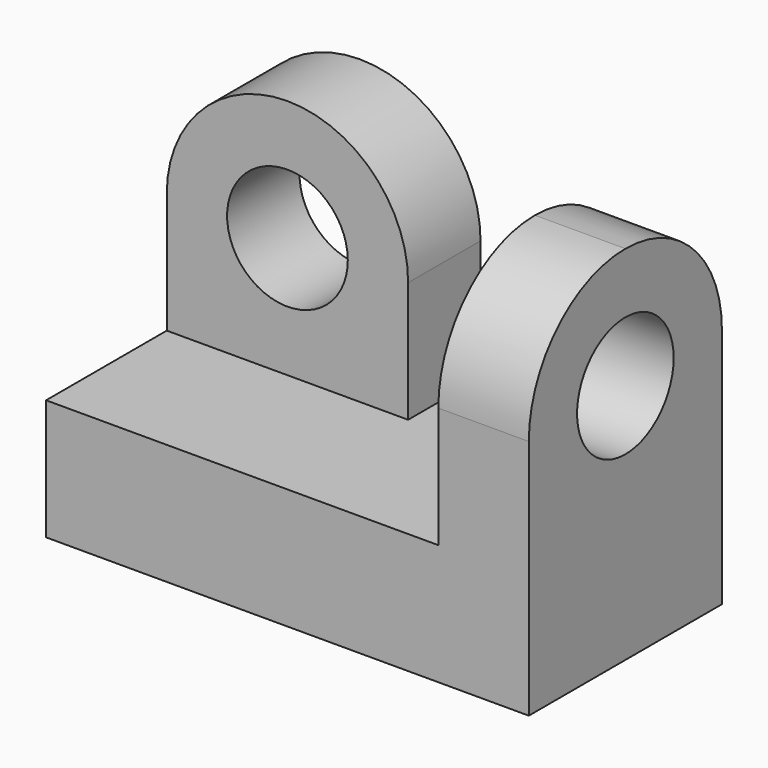
from build123d import *

# Parameters (mm, degrees)
F1_DEPTH = 40
F0_R     = 10
F2_DEPTH = 15
F4_R     = 19.99999
F5_R     = 10
F6_DEPTH = 15


# Not quite as in the source:
# - a fillet or chamfer is up to 0.001 mm smaller than in the source, because OpenCascade refuses the exact size


with BuildPart() as f1:
    # F0 (on Front) → F1 (new body)
    with BuildSketch(Plane.XZ):
        Polygon((0, 20), (0, 0), (80, 0), (80, 60), (65, 60), (65, 20), (40, 20), align=None)
    extrude(amount=F1_DEPTH)

    # F0 (on Front) → F2 (join)
    with BuildSketch(Plane.XZ):
        with BuildLine():
            Line((0, 40), (0, 20))
            Line((0, 20), (40, 20))
            Line((40, 20), (40, 40))
            ThreePointArc((40, 40), (20, 60), (0, 40))
        make_face()
        with Locations((20, 40)):
            Circle(F0_R, mode=Mode.SUBTRACT)
    extrude(amount=F2_DEPTH)

    # F4 (radius 20 in the source; OpenCascade refuses exactly that, so slightly less here)
    f4_edges = [f1.edges().sort_by_distance(p)[0] for p in [
        (72.5, -40, 60),
        (72.5, 0, 60),
    ]]
    fillet(f4_edges, radius=F4_R)

    # F5 (on face) → F6 (cut, through all)
    with BuildSketch(Plane.YZ.offset(80)):
        with Locations((-20, 40)):
            Circle(F5_R)
    extrude(amount=-F6_DEPTH, mode=Mode.SUBTRACT)


solid = f1.part
